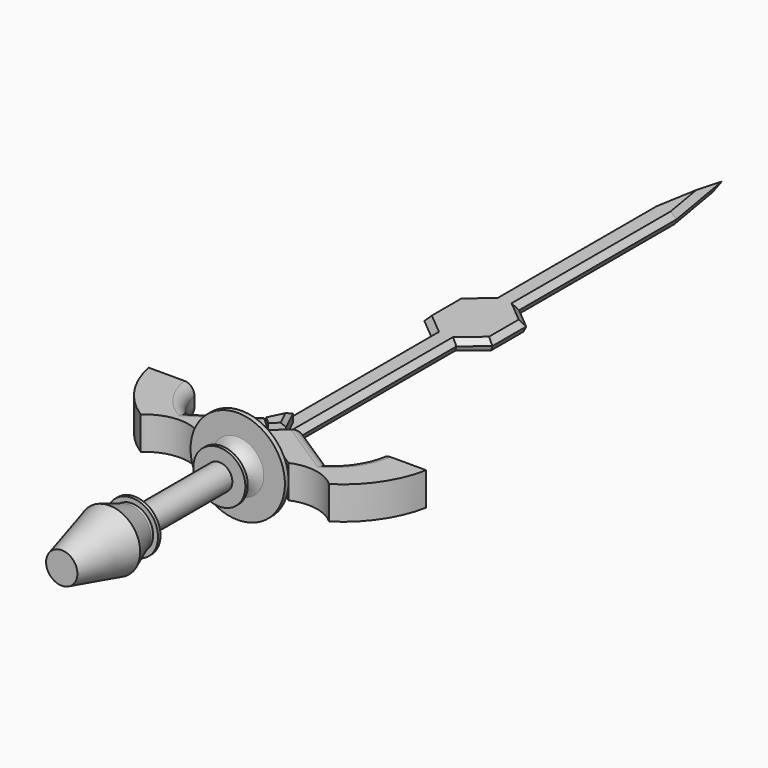
from build123d import *

# Parameters (mm, degrees)
F0_W          = 7.8241664692
F0_H          = 1.0562075689
F0_W_2        = 4.8171242003
F0_H_2        = 39.2373276583
F2_DEPTH      = 6.096
F3_DEPTH      = 8.382
F4_SIZE       = 1.524
F5_DEPTH      = 3.81
F6_T1_DEPTH   = 97.5220461555
F6_T3_DEPTH   = 97.5220461555
F6_T5_DEPTH   = 44.6077719326
F6_T10_DEPTH  = 123.8581218987
F6_T15_DEPTH  = 123.8581218987
F6_T20_DEPTH  = 36.5295973116
F6_T25_DEPTH  = 36.5295973116
F6_T30_DEPTH  = 99.0078726059
F6_T37_DEPTH  = 99.0078726059
F6_T44_DEPTH  = 99.0078726059
F6_T51_DEPTH  = 99.0078726059
F6_T58_DEPTH  = 36.5295973116
F6_T63_DEPTH  = 36.5295973116
F6_T69_DEPTH  = 123.8581218987
F6_T73_DEPTH  = 36.5295973116
F6_T80_DEPTH  = 36.5295973116
F6_T84_DEPTH  = 123.8581218987
F6_T91_DEPTH  = 36.5295973116
F6_T95_DEPTH  = 99.0078726059
F6_T102_DEPTH = 99.0078726059
F6_T106_DEPTH = 36.5295973116
F7_SIZE       = 2.54
F8_R          = 3.6792614691
F9_T3_DEPTH   = 46.9050816296
F9_S5_R       = 21.1572469119
F9_T6_DEPTH   = 27
F9_T9_DEPTH   = 46.9050816296
F9_S10_R      = 21.1572469119
F9_T11_DEPTH  = 27
F9_T15_ANGLE  = 113.8337050243
F9_T19_ANGLE  = 113.8337050243
F9_T24_ANGLE  = 113.8337050243
F9_T28_DEPTH  = 46.9050816296
F9_S29_R      = 21.1572469119
F9_T30_DEPTH  = 27
F9_T35_DEPTH  = 46.9050816296
F9_S36_R      = 21.1572469119
F9_T37_DEPTH  = 27
F9_T40_ANGLE  = 113.8337050243
F10_SIZE      = 1.524


# Not quite as in the source:
# - a fillet or chamfer that OpenCascade refuses, or shapes differently, is made with other operations: its cross-section is extruded or revolved along the edge and cut away or added


with BuildPart() as f1:
    # F0 (on Top) → F1 (revolve)
    with BuildSketch(Plane.XY):
        Polygon((0, -34.161419578), (-11.372709382, -34.161419578), (-5.7964275313, -56.2130698955), (0, -56.2130698955), align=None)
        Polygon((-7.8241664692, -24.7831277904), (-11.372709382, -34.161419578), (0, -34.161419578), (0, -24.7831277904), align=None)
        with Locations((-3.9120832346, -24.2550240059)):
            Rectangle(F0_W, F0_H)
        Polygon((-9.6342484006, -23.7269202215), (-7.8241664692, -23.7269202215), (0, -23.7269202215), (0, -22.5793192292), (-4.8171242003, -22.5793192292), (-9.6342484006, -22.5793192292), align=None)
        with Locations((-2.4085621002, -2.9606554001)):
            Rectangle(F0_W_2, F0_H_2)
        Polygon((-4.8171242003, 16.6580084291), (0, 16.6580084291), (0, 17.7766310833), (-4.8171242003, 17.7766310833), (-9.6342484006, 17.7766310833), (-9.6342484006, 16.6580084291), align=None)
        with BuildLine():
            Line((-4.8171242003, 17.7766310833), (0, 17.7766310833))
            Line((0, 17.7766310833), (0, 25.1468530215))
            Line((0, 25.1468530215), (-9.6342484006, 25.1468530215))
            ThreePointArc((-9.6342484006, 25.1468530215), (-5.9683103375, 22.283553964), (-4.8171242003, 17.7766310833))
        make_face()
        Polygon((-9.6342484006, 25.1468530215), (0, 25.1468530215), (0, 26.8842804851), (-15.5501095578, 26.8842804851), (-17.4540731808, 26.8842804851), (-17.4540731808, 25.1468530215), align=None)
        Polygon((-17.4540731808, 26.8842804851), (-15.5501095578, 26.8842804851), (-5.9436, 34.0511790619), align=None)
    revolve(axis=Axis((0, -40.4980988429, 0), (0, -1, 0)))


with BuildPart() as f2:
    # F0 (on Top) → F2 (new body, symmetric)
    with BuildSketch(Plane.XY):
        with BuildLine():
            Line((-5.9436, 34.0511790619), (0, 34.0511790619))
            Line((0, 34.0511790619), (5.9436, 34.0511790619))
            Line((5.9436, 34.0511790619), (17.4540731808, 26.8842804851))
            ThreePointArc((17.4540731808, 26.8842804851), (26.5904955681, 27.931291107), (34.8283770844, 23.8437792226))
            ThreePointArc((34.8283770844, 23.8437792226), (45.592031181, 34.301992079), (51.3339626832, 48.1678021269))
            Line((51.3339626832, 48.1678021269), (34.394017932, 48.1678021269))
            ThreePointArc((34.394017932, 48.1678021269), (31.4125070828, 40.4618684875), (25.7068659801, 34.4855418728))
            Line((25.7068659801, 34.4855418728), (7.6810297501, 46.2131914286))
            Line((7.6810297501, 46.2131914286), (3.8405148751, 42.7383310137))
            Line((3.8405148751, 42.7383310137), (0, 39.2634705988))
            Line((0, 39.2634705988), (-3.8405148751, 42.7383310137))
            Line((-3.8405148751, 42.7383310137), (-7.6810297501, 46.2131914286))
            Line((-7.6810297501, 46.2131914286), (-25.7068659801, 34.4855418728))
            ThreePointArc((-25.7068659801, 34.4855418728), (-31.4125070828, 40.4618684875), (-34.394017932, 48.1678021269))
            Line((-34.394017932, 48.1678021269), (-51.3339626832, 48.1678021269))
            ThreePointArc((-51.3339626832, 48.1678021269), (-45.592031181, 34.301992079), (-34.8283770844, 23.8437792226))
            ThreePointArc((-34.8283770844, 23.8437792226), (-26.5904955681, 27.931291107), (-17.4540731808, 26.8842804851))
            Line((-17.4540731808, 26.8842804851), (-5.9436, 34.0511790619))
        make_face()
    extrude(amount=F2_DEPTH, both=True)

    # F0 (on Top) → F3 (join, symmetric)
    with BuildSketch(Plane.XY):
        Polygon((0, 42.7383310137), (-3.8405148751, 42.7383310137), (0, 39.2634705988), align=None)
        Polygon((3.8405148751, 42.7383310137), (0, 50.6857074797), (0, 42.7383310137), align=None)
        Polygon((0, 42.7383310137), (0, 39.2634705988), (3.8405148751, 42.7383310137), align=None)
        Polygon((0, 50.6857074797), (-3.8405148751, 42.7383310137), (0, 42.7383310137), align=None)
    extrude(amount=F3_DEPTH, both=True)

    # F4
    f4_edges = [f2.edges().sort_by_distance(p)[0] for p in [
        (-1.920257, 46.712019, 8.382),
        (1.920257, 46.712019, 8.382),
    ]]
    chamfer(f4_edges, length=F4_SIZE)

    # F0 (on Top) → F5 (join)
    with BuildSketch(Plane.XY):
        Polygon((-7.6810297501, 119.0927648767), (-7.6810297501, 46.2131914286), (-3.8405148751, 42.7383310137), (0, 50.6857074797), (3.8405148751, 42.7383310137), (7.6810297501, 46.2131914286), (7.6810297501, 119.0927648767), (15.6595040762, 125.7659163596), (15.6595040762, 144.2453891344), (7.6810297501, 150.9185406173), (7.6810297501, 222.5200642005), (0, 267.129060492), (-7.6810297501, 222.5200642005), (-7.6810297501, 150.9185406173), (-15.6595040762, 144.2453891344), (-15.6595040762, 125.7659163596), align=None)
    extrude(amount=F5_DEPTH)

    # F6: chamfer of 5.08 on 12 edges, made by hand

    # F6_s2 → F6_t1 (cut)
    with BuildSketch(Plane(origin=(46.8882194732, 272.3119785546, 0), x_dir=(0, 0, 1), z_dir=(-0.169688584, -0.9854977344, 0))):
        Polygon((3.81, 40.2487520321), (-1.27, 45.3287520321), (3.81, 45.3287520321), align=None)
    extrude(amount=F6_T1_DEPTH, mode=Mode.SUBTRACT)

    # F6_s4 → F6_t3 (cut)
    with BuildSketch(Plane(origin=(-30.3398415479, 176.2042230174, 0), x_dir=(0, 0, 1), z_dir=(-0.169688584, 0.9854977344, 0))):
        Polygon((3.81, 40.2487520321), (-1.27, 45.3287520321), (3.81, 45.3287520321), align=None)
    extrude(amount=F6_T3_DEPTH, mode=Mode.SUBTRACT)

    # F6_s6 → F6_t5 (cut)
    with BuildSketch(Plane.XZ.offset(-157.3095387133)):
        Polygon((-10.5795040762, 3.81), (-15.6595040762, -1.27), (-15.6595040762, 3.81), align=None)
        Polygon((10.5795040762, 3.81), (15.6595040762, -1.27), (15.6595040762, 3.81), align=None)
    extrude(amount=F6_T5_DEPTH, mode=Mode.SUBTRACT)


with BuildPart() as f6_tool8:
    # F6_s9 → F6_t10 (new body)
    with BuildSketch(Plane.XZ.offset(-261.7125129371)):
        Polygon((-2.6010297501, 3.81), (-7.6810297501, -1.27), (-7.6810297501, 3.81), align=None)
    extrude(amount=F6_T10_DEPTH)

    split(bisect_by=Plane(origin=(-77.4324365441, 92.5788525195, 0), x_dir=(0, 0, 1), z_dir=(-0.6415690988, 0.7670652459, 0)), keep=Keep.TOP)


with BuildPart() as f2_1:
    add(f2.part)

    # F6_t7: cut F6_tool8
    add(f6_tool8.part, mode=Mode.SUBTRACT)


with BuildPart() as f6_tool13:
    # F6_s14 → F6_t15 (new body)
    with BuildSketch(Plane.XZ.offset(-137.8543910384)):
        Polygon((2.6010297501, 3.81), (7.6810297501, -1.27), (7.6810297501, 3.81), align=None)
    extrude(amount=-F6_T15_DEPTH)

    split(bisect_by=Plane(origin=(77.4324365441, 92.5788525195, 0), x_dir=(0, 0, 1), z_dir=(0.6415690988, 0.7670652459, 0)), keep=Keep.TOP)


with BuildPart() as f2_2:
    add(f2_1.part)

    # F6_t12: cut F6_tool13
    add(f6_tool13.part, mode=Mode.SUBTRACT)


with BuildPart() as f6_tool18:
    # F6_s19 → F6_t20 (new body)
    with BuildSketch(Plane(origin=(79.7724619032, 66.7212427697, 0), x_dir=(0, 0, 1), z_dir=(-0.7670652459, -0.6415690988, 0))):
        Polygon((3.81, 115.6122788043), (-1.27, 120.6922788043), (3.81, 120.6922788043), align=None)
    extrude(amount=F6_T20_DEPTH)

    split(bisect_by=Plane.YZ.offset(-7.6810297501), keep=Keep.BOTTOM)


with BuildPart() as f2_3:
    add(f2_2.part)

    # F6_t17: cut F6_tool18
    add(f6_tool18.part, mode=Mode.SUBTRACT)


with BuildPart() as f6_tool23:
    # F6_s24 → F6_t25 (new body)
    with BuildSketch(Plane(origin=(-81.1275331649, 67.8546168247, 0), x_dir=(0, 0, 1), z_dir=(0.7670652459, -0.6415690988, 0))):
        Polygon((3.81, -91.5040096406), (-1.27, -86.4240096406), (3.81, -86.4240096406), align=None)
    extrude(amount=F6_T25_DEPTH)

    split(bisect_by=Plane.YZ.offset(-7.6810297501), keep=Keep.BOTTOM)


with BuildPart() as f2_4:
    add(f2_3.part)

    # F6_t22: cut F6_tool23
    add(f6_tool23.part, mode=Mode.SUBTRACT)


with BuildPart() as f6_tool28:
    # F6_s29 → F6_t30 (new body)
    with BuildSketch(Plane.XZ.offset(-132.1569144556)):
        Polygon((-2.6010297501, 3.81), (-7.6810297501, -1.27), (-7.6810297501, 3.81), align=None)
    extrude(amount=F6_T30_DEPTH)

    split(bisect_by=Plane(origin=(19.5338824426, 21.5894042153, 0), x_dir=(0, 0, 1), z_dir=(0.6709248817, 0.741525322, 0)), keep=Keep.TOP)

    split(bisect_by=Plane(origin=(-23.4090135534, 35.980529825, 0), x_dir=(0, 0, 1), z_dir=(-0.5453431779, 0.8382128718, 0)), keep=Keep.TOP)

    split(bisect_by=Plane(origin=(55.4469739795, 66.2928542068, 0), x_dir=(0, 0, 1), z_dir=(-0.6415690988, -0.7670652459, 0)), keep=Keep.TOP)


with BuildPart() as f2_5:
    add(f2_4.part)

    # F6_t27: cut F6_tool28
    add(f6_tool28.part, mode=Mode.SUBTRACT)


with BuildPart() as f6_tool35:
    # F6_s36 → F6_t37 (new body)
    with BuildSketch(Plane.XZ.offset(-132.1569144556)):
        Polygon((-2.6010297501, 3.81), (-7.6810297501, -1.27), (-7.6810297501, 3.81), align=None)
    extrude(amount=F6_T37_DEPTH)

    split(bisect_by=Plane(origin=(-19.8565416293, 9.5955368191, 0), x_dir=(0, 0, 1), z_dir=(-0.9003807807, 0.4351028036, 0)), keep=Keep.TOP)

    split(bisect_by=Plane(origin=(19.5338824426, 21.5894042153, 0), x_dir=(0, 0, 1), z_dir=(0.6709248817, 0.741525322, 0)), keep=Keep.TOP)

    split(bisect_by=Plane(origin=(-23.4090135534, 35.980529825, 0), x_dir=(0, 0, 1), z_dir=(0.5453431779, -0.8382128718, 0)), keep=Keep.TOP)


with BuildPart() as f2_6:
    add(f2_5.part)

    # F6_t34: cut F6_tool35
    add(f6_tool35.part, mode=Mode.SUBTRACT)


with BuildPart() as f6_tool42:
    # F6_s43 → F6_t44 (new body)
    with BuildSketch(Plane.XZ.offset(-33.1490418497)):
        Polygon((2.6010297501, 3.81), (7.6810297501, -1.27), (7.6810297501, 3.81), align=None)
    extrude(amount=-F6_T44_DEPTH)

    split(bisect_by=Plane(origin=(19.8565416293, 9.5955368191, 0), x_dir=(0, 0, 1), z_dir=(0.9003807807, 0.4351028036, 0)), keep=Keep.TOP)

    split(bisect_by=Plane(origin=(-19.5338824426, 21.5894042153, 0), x_dir=(0, 0, 1), z_dir=(-0.6709248817, 0.741525322, 0)), keep=Keep.TOP)

    split(bisect_by=Plane(origin=(23.4090135534, 35.980529825, 0), x_dir=(0, 0, 1), z_dir=(-0.5453431779, -0.8382128718, 0)), keep=Keep.TOP)


with BuildPart() as f2_7:
    add(f2_6.part)

    # F6_t41: cut F6_tool42
    add(f6_tool42.part, mode=Mode.SUBTRACT)


with BuildPart() as f6_tool49:
    # F6_s50 → F6_t51 (new body)
    with BuildSketch(Plane.XZ.offset(-33.1490418497)):
        Polygon((2.6010297501, 3.81), (7.6810297501, -1.27), (7.6810297501, 3.81), align=None)
    extrude(amount=-F6_T51_DEPTH)

    split(bisect_by=Plane(origin=(-19.5338824426, 21.5894042153, 0), x_dir=(0, 0, 1), z_dir=(-0.6709248817, 0.741525322, 0)), keep=Keep.TOP)

    split(bisect_by=Plane(origin=(23.4090135534, 35.980529825, 0), x_dir=(0, 0, 1), z_dir=(0.5453431779, 0.8382128718, 0)), keep=Keep.TOP)

    split(bisect_by=Plane(origin=(-55.4469739795, 66.2928542068, 0), x_dir=(0, 0, 1), z_dir=(0.6415690988, -0.7670652459, 0)), keep=Keep.TOP)


with BuildPart() as f2_8:
    add(f2_7.part)

    # F6_t48: cut F6_tool49
    add(f6_tool49.part, mode=Mode.SUBTRACT)


with BuildPart() as f6_tool56:
    # F6_s57 → F6_t58 (new body)
    with BuildSketch(Plane(origin=(53.1069486204, 44.4183559981, 0), x_dir=(0, 0, 1), z_dir=(0.7670652459, 0.6415690988, 0))):
        Polygon((3.81, -91.5040096406), (-1.27, -86.4240096406), (3.81, -86.4240096406), align=None)
    extrude(amount=F6_T58_DEPTH)

    split(bisect_by=Plane.YZ.offset(7.6810297501), keep=Keep.TOP)


with BuildPart() as f2_9:
    add(f2_8.part)

    # F6_t55: cut F6_tool56
    add(f6_tool56.part, mode=Mode.SUBTRACT)


with BuildPart() as f6_tool61:
    # F6_s62 → F6_t63 (new body)
    with BuildSketch(Plane(origin=(-51.7518773587, 43.2849819431, 0), x_dir=(0, 0, 1), z_dir=(-0.7670652459, 0.6415690988, 0))):
        Polygon((3.81, 115.6122788043), (-1.27, 120.6922788043), (3.81, 120.6922788043), align=None)
    extrude(amount=F6_T63_DEPTH)

    split(bisect_by=Plane.YZ.offset(7.6810297501), keep=Keep.TOP)


with BuildPart() as f2_10:
    add(f2_9.part)

    # F6_t60: cut F6_tool61
    add(f6_tool61.part, mode=Mode.SUBTRACT)


with BuildPart() as f6_tool67:
    # F6_s68 → F6_t69 (new body)
    with BuildSketch(Plane.XZ.offset(-261.7125129371)):
        Polygon((-2.6010297501, 3.81), (-7.6810297501, -1.27), (-7.6810297501, 3.81), align=None)
    extrude(amount=F6_T69_DEPTH)

    split(bisect_by=Plane(origin=(-77.4324365441, 92.5788525195, 0), x_dir=(0, 0, 1), z_dir=(0.6415690988, -0.7670652459, 0)), keep=Keep.TOP)


with BuildPart() as f6_tool71:
    # F6_s72 → F6_t73 (new body)
    with BuildSketch(Plane(origin=(79.7724619032, 66.7212427697, 0), x_dir=(0, 0, 1), z_dir=(-0.7670652459, -0.6415690988, 0))):
        Polygon((3.81, 115.6122788043), (-1.27, 120.6922788043), (3.81, 120.6922788043), align=None)
    extrude(amount=F6_T73_DEPTH)

    split(bisect_by=Plane.YZ.offset(-7.6810297501), keep=Keep.TOP)


with BuildPart() as f6_tool67_1:
    add(f6_tool67.part)

    # F6_t75: intersect F6_tool71
    add(f6_tool71.part, mode=Mode.INTERSECT)


with BuildPart() as f2_11:
    add(f2_10.part)

    # F6_t65: cut F6_tool67
    add(f6_tool67_1.part, mode=Mode.SUBTRACT)


with BuildPart() as f6_tool78:
    # F6_s79 → F6_t80 (new body)
    with BuildSketch(Plane(origin=(-51.7518773587, 43.2849819431, 0), x_dir=(0, 0, 1), z_dir=(-0.7670652459, 0.6415690988, 0))):
        Polygon((3.81, 115.6122788043), (-1.27, 120.6922788043), (3.81, 120.6922788043), align=None)
    extrude(amount=F6_T80_DEPTH)

    split(bisect_by=Plane.YZ.offset(7.6810297501), keep=Keep.BOTTOM)


with BuildPart() as f6_tool82:
    # F6_s83 → F6_t84 (new body)
    with BuildSketch(Plane.XZ.offset(-137.8543910384)):
        Polygon((2.6010297501, 3.81), (7.6810297501, -1.27), (7.6810297501, 3.81), align=None)
    extrude(amount=-F6_T84_DEPTH)

    split(bisect_by=Plane(origin=(77.4324365441, 92.5788525195, 0), x_dir=(0, 0, 1), z_dir=(-0.6415690988, -0.7670652459, 0)), keep=Keep.TOP)


with BuildPart() as f6_tool78_1:
    add(f6_tool78.part)

    # F6_t86: intersect F6_tool82
    add(f6_tool82.part, mode=Mode.INTERSECT)


with BuildPart() as f2_12:
    add(f2_11.part)

    # F6_t76: cut F6_tool78
    add(f6_tool78_1.part, mode=Mode.SUBTRACT)


with BuildPart() as f6_tool89:
    # F6_s90 → F6_t91 (new body)
    with BuildSketch(Plane(origin=(-81.1275331649, 67.8546168247, 0), x_dir=(0, 0, 1), z_dir=(0.7670652459, -0.6415690988, 0))):
        Polygon((3.81, -91.5040096406), (-1.27, -86.4240096406), (3.81, -86.4240096406), align=None)
    extrude(amount=F6_T91_DEPTH)

    split(bisect_by=Plane.YZ.offset(-7.6810297501), keep=Keep.TOP)


with BuildPart() as f6_tool93:
    # F6_s94 → F6_t95 (new body)
    with BuildSketch(Plane.XZ.offset(-132.1569144556)):
        Polygon((-2.6010297501, 3.81), (-7.6810297501, -1.27), (-7.6810297501, 3.81), align=None)
    extrude(amount=F6_T95_DEPTH)

    split(bisect_by=Plane(origin=(55.4469739795, 66.2928542068, 0), x_dir=(0, 0, 1), z_dir=(0.6415690988, 0.7670652459, 0)), keep=Keep.TOP)


with BuildPart() as f6_tool89_1:
    add(f6_tool89.part)

    # F6_t97: intersect F6_tool93
    add(f6_tool93.part, mode=Mode.INTERSECT)


with BuildPart() as f2_13:
    add(f2_12.part)

    # F6_t87: cut F6_tool89
    add(f6_tool89_1.part, mode=Mode.SUBTRACT)


with BuildPart() as f6_tool100:
    # F6_s101 → F6_t102 (new body)
    with BuildSketch(Plane.XZ.offset(-33.1490418497)):
        Polygon((2.6010297501, 3.81), (7.6810297501, -1.27), (7.6810297501, 3.81), align=None)
    extrude(amount=-F6_T102_DEPTH)

    split(bisect_by=Plane(origin=(-55.4469739795, 66.2928542068, 0), x_dir=(0, 0, 1), z_dir=(-0.6415690988, 0.7670652459, 0)), keep=Keep.TOP)


with BuildPart() as f6_tool104:
    # F6_s105 → F6_t106 (new body)
    with BuildSketch(Plane(origin=(53.1069486204, 44.4183559981, 0), x_dir=(0, 0, 1), z_dir=(0.7670652459, 0.6415690988, 0))):
        Polygon((3.81, -91.5040096406), (-1.27, -86.4240096406), (3.81, -86.4240096406), align=None)
    extrude(amount=F6_T106_DEPTH)

    split(bisect_by=Plane.YZ.offset(7.6810297501), keep=Keep.BOTTOM)


with BuildPart() as f6_tool100_1:
    add(f6_tool100.part)

    # F6_t108: intersect F6_tool104
    add(f6_tool104.part, mode=Mode.INTERSECT)


with BuildPart() as f2_14:
    add(f2_13.part)

    # F6_t98: cut F6_tool100
    add(f6_tool100_1.part, mode=Mode.SUBTRACT)

    # F7
    f7_edges = [f2_14.edges().sort_by_distance(p)[0] for p in [
        (14.389504, 135.005653, 0),
        (10.400267, 123.022781, 0),
        (10.400267, 146.988525, 0),
        (-14.389504, 135.005653, 0),
        (-10.400267, 146.988525, 0),
        (-10.400267, 123.022781, 0),
        (6.41103, 82.375156, 0),
        (-6.41103, 82.375156, 0),
        (6.41103, 186.368313, 0),
        (-6.41103, 186.368313, 0),
        (3.205515, 241.028143, 0),
        (-3.205515, 241.028143, 0),
    ]]
    chamfer(f7_edges, length=F7_SIZE)

    # F8
    f8_edges = [f2_14.edges().sort_by_distance(p)[0] for p in [
        (-16.693948, 40.349367, 6.096),
        (16.693948, 40.349367, 6.096),
        (31.412507, 40.461868, 6.096),
        (-31.412507, 40.461868, 6.096),
    ]]
    fillet(f8_edges, radius=F8_R)

    # F9: fillet of radius 5.08 on 4 edges, made by hand


with BuildPart() as f9_tool1:
    # F9_s2 → F9_t3 (new body)
    with BuildSketch(Plane(origin=(12.943155898, -8.4208463109, 0), x_dir=(0, 0, 1), z_dir=(-0.8382128718, 0.5453431779, 0))):
        with BuildLine():
            ThreePointArc((-6.096, 37.8452890733), (-4.6081024484, 41.4373915217), (-1.016, 42.9252890733))
            Line((-1.016, 42.9252890733), (-6.096, 42.9252890733))
            Line((-6.096, 42.9252890733), (-6.096, 37.8452890733))
        make_face()
    extrude(amount=F9_T3_DEPTH)

    split(bisect_by=Plane(origin=(-19.5338824426, 21.5894042153, 0), x_dir=(0, 0, 1), z_dir=(0.6709248817, -0.741525322, 0)), keep=Keep.TOP)

    # F9_s5 → F9_t6 (intersect, symmetric)
    with BuildSketch(Plane.XY.offset(-3.6)):
        with Locations((13.5512896309, 51.8023273859)):
            Circle(F9_S5_R)
    extrude(amount=F9_T6_DEPTH, both=True, mode=Mode.INTERSECT)


with BuildPart() as f9_tool7:
    # F9_s8 → F9_t9 (new body)
    with BuildSketch(Plane(origin=(26.3732872745, 17.1585199623, 0), x_dir=(0, 0, 1), z_dir=(-0.8382128718, -0.5453431779, 0))):
        with BuildLine():
            ThreePointArc((-1.016, 42.9252890733), (-4.6081024484, 41.4373915217), (-6.096, 37.8452890733))
            Line((-6.096, 37.8452890733), (-6.096, 42.9252890733))
            Line((-6.096, 42.9252890733), (-1.016, 42.9252890733))
        make_face()
    extrude(amount=F9_T9_DEPTH)

    # F9_s10 → F9_t11 (intersect, symmetric)
    with BuildSketch(Plane.XY.offset(-3.6)):
        with Locations((-13.5512896309, 51.8023273859)):
            Circle(F9_S10_R)
    extrude(amount=F9_T11_DEPTH, both=True, mode=Mode.INTERSECT)

    split(bisect_by=Plane(origin=(19.5338824426, 21.5894042153, 0), x_dir=(0, 0, 1), z_dir=(-0.6709248817, -0.741525322, 0)), keep=Keep.TOP)


with BuildPart() as f9_tool13:
    # F9_s14 → F9_t15 (revolve)
    with BuildSketch(Plane(origin=(-17.2193160086, 37.77641099, 0), x_dir=(0, 0, 1), z_dir=(-0.4147653159, 0.9099284217, 0))):
        with BuildLine():
            ThreePointArc((-6.096, 60.0537591828), (-4.6081024484, 56.4616567344), (-1.016, 54.9737591828))
            Line((-1.016, 54.9737591828), (-6.096, 54.9737591828))
            Line((-6.096, 54.9737591828), (-6.096, 60.0537591828))
        make_face()
    revolve(axis=Axis((13.5512896309, 51.8023273859, -6.096), (0, 0, -1)), revolution_arc=F9_T15_ANGLE)

    split(bisect_by=Plane(origin=(23.4090135534, 35.980529825, 0), x_dir=(0, 0, 1), z_dir=(0.5453431779, 0.8382128718, 0)), keep=Keep.TOP)


with BuildPart() as f9_tool17:
    # F9_s18 → F9_t19 (revolve)
    with BuildSketch(Plane(origin=(-14.1558910975, 0.1657482479, 0), x_dir=(0, 0, 1), z_dir=(0.9999314593, -0.0117079798, 0))):
        with BuildLine():
            ThreePointArc((-6.096, -25.4028716783), (-4.6081024484, -28.9949741268), (-1.016, -30.4828716783))
            Line((-1.016, -30.4828716783), (-6.096, -30.4828716783))
            Line((-6.096, -30.4828716783), (-6.096, -25.4028716783))
        make_face()
    revolve(axis=Axis((-13.5512896309, 51.8023273859, -6.096), (0, 0, -1)), revolution_arc=F9_T19_ANGLE)

    split(bisect_by=Plane(origin=(-23.4090135534, 35.980529825, 0), x_dir=(0, 0, 1), z_dir=(-0.5453431779, 0.8382128718, 0)), keep=Keep.TOP)


with BuildPart() as f9_tool22:
    # F9_s23 → F9_t24 (revolve)
    with BuildSketch(Plane(origin=(-17.2193160086, 37.77641099, 0), x_dir=(0, 0, 1), z_dir=(-0.4147653159, 0.9099284217, 0))):
        with BuildLine():
            ThreePointArc((-6.096, 60.0537591828), (-4.6081024484, 56.4616567344), (-1.016, 54.9737591828))
            Line((-1.016, 54.9737591828), (-6.096, 54.9737591828))
            Line((-6.096, 54.9737591828), (-6.096, 60.0537591828))
        make_face()
    revolve(axis=Axis((13.5512896309, 51.8023273859, -6.096), (0, 0, -1)), revolution_arc=F9_T24_ANGLE)

    split(bisect_by=Plane(origin=(23.4090135534, 35.980529825, 0), x_dir=(0, 0, 1), z_dir=(-0.5453431779, -0.8382128718, 0)), keep=Keep.TOP)


with BuildPart() as f9_tool26:
    # F9_s27 → F9_t28 (new body)
    with BuildSketch(Plane(origin=(12.943155898, -8.4208463109, 0), x_dir=(0, 0, 1), z_dir=(-0.8382128718, 0.5453431779, 0))):
        with BuildLine():
            ThreePointArc((-6.096, 37.8452890733), (-4.6081024484, 41.4373915217), (-1.016, 42.9252890733))
            Line((-1.016, 42.9252890733), (-6.096, 42.9252890733))
            Line((-6.096, 42.9252890733), (-6.096, 37.8452890733))
        make_face()
    extrude(amount=F9_T28_DEPTH)

    # F9_s29 → F9_t30 (cut, symmetric)
    with BuildSketch(Plane.XY.offset(-3.6)):
        with Locations((13.5512896309, 51.8023273859)):
            Circle(F9_S29_R)
    extrude(amount=F9_T30_DEPTH, both=True, mode=Mode.SUBTRACT)


with BuildPart() as f9_tool22_1:
    add(f9_tool22.part)

    # F9_t31: intersect F9_tool26
    add(f9_tool26.part, mode=Mode.INTERSECT)


with BuildPart() as f9_tool33:
    # F9_s34 → F9_t35 (new body)
    with BuildSketch(Plane(origin=(26.3732872745, 17.1585199623, 0), x_dir=(0, 0, 1), z_dir=(-0.8382128718, -0.5453431779, 0))):
        with BuildLine():
            ThreePointArc((-1.016, 42.9252890733), (-4.6081024484, 41.4373915217), (-6.096, 37.8452890733))
            Line((-6.096, 37.8452890733), (-6.096, 42.9252890733))
            Line((-6.096, 42.9252890733), (-1.016, 42.9252890733))
        make_face()
    extrude(amount=F9_T35_DEPTH)

    # F9_s36 → F9_t37 (cut, symmetric)
    with BuildSketch(Plane.XY.offset(-3.6)):
        with Locations((-13.5512896309, 51.8023273859)):
            Circle(F9_S36_R)
    extrude(amount=F9_T37_DEPTH, both=True, mode=Mode.SUBTRACT)


with BuildPart() as f9_tool38:
    # F9_s39 → F9_t40 (revolve)
    with BuildSketch(Plane(origin=(-14.1558910975, 0.1657482479, 0), x_dir=(0, 0, 1), z_dir=(0.9999314593, -0.0117079798, 0))):
        with BuildLine():
            ThreePointArc((-6.096, -25.4028716783), (-4.6081024484, -28.9949741268), (-1.016, -30.4828716783))
            Line((-1.016, -30.4828716783), (-6.096, -30.4828716783))
            Line((-6.096, -30.4828716783), (-6.096, -25.4028716783))
        make_face()
    revolve(axis=Axis((-13.5512896309, 51.8023273859, -6.096), (0, 0, -1)), revolution_arc=F9_T40_ANGLE)

    split(bisect_by=Plane(origin=(-23.4090135534, 35.980529825, 0), x_dir=(0, 0, 1), z_dir=(0.5453431779, -0.8382128718, 0)), keep=Keep.TOP)


with BuildPart() as f9_tool33_1:
    add(f9_tool33.part)

    # F9_t42: intersect F9_tool38
    add(f9_tool38.part, mode=Mode.INTERSECT)


with BuildPart() as f2_15:
    add(f2_14.part)

    # F9_t43: cut F9_tool1, F9_tool7, F9_tool13, F9_tool17, F9_tool22, F9_tool33
    add([f9_tool1.part, f9_tool7.part, f9_tool13.part, f9_tool17.part, f9_tool22_1.part, f9_tool33_1.part], mode=Mode.SUBTRACT)

    # F10
    f10_edges = [f2_15.edges().sort_by_distance(p)[0] for p in [
        (1.920257, 46.712019, -8.382),
        (-1.920257, 46.712019, -8.382),
    ]]
    chamfer(f10_edges, length=F10_SIZE)


solid = Compound([f1.part, f2_15.part])
